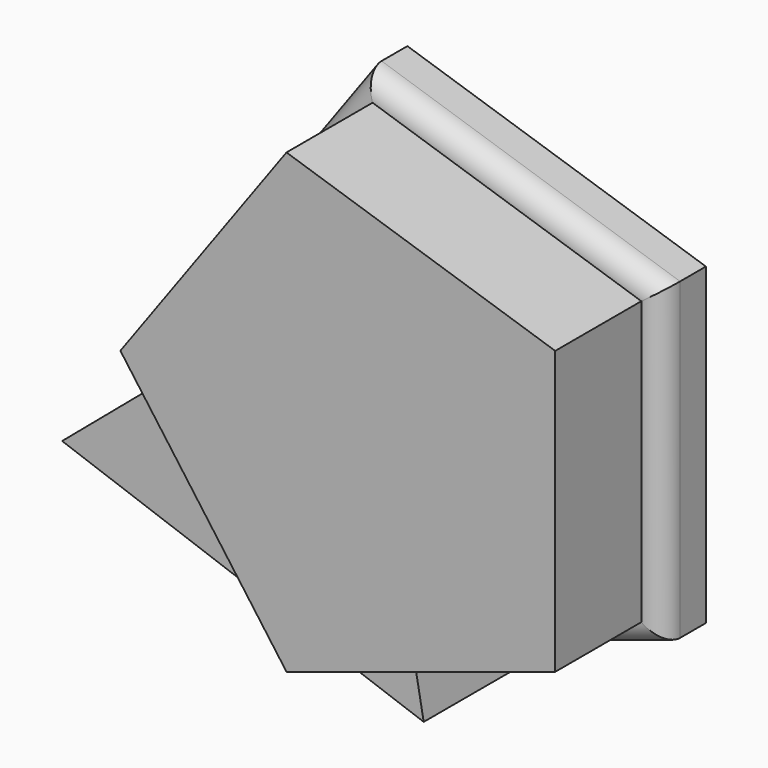
from build123d import *

# Parameters (mm, degrees)
F1_DEPTH     = 12.7
F2_R         = 5.08
F3_TEXT_SIZE = 35.0921052612
F4_DEPTH     = 25.4
F6_DEPTH     = 25.4


# Not quite as in the source:
# - Text() gives the source's letters only with a copy of the font that has no kerning and outlines rounded to 1/6400 em; it was checked with that copy


with BuildPart() as f1:
    # F0 (on Front) → F1 (new body)
    with BuildSketch(Plane.XZ):
        Polygon((50.9689189494, -37.0310872232), (50.9689189494, 37.0310872232), (-19.4683946688, 59.9175577675), (-63.0010485611, 0), (-19.4683946688, -59.9175577675), align=None)
    extrude(amount=F1_DEPTH)

    # F2
    f2_edges = [f1.edges().sort_by_distance(p)[0] for p in [
        (15.750262, -12.7, -48.474322),
        (50.968919, -12.7, 0),
        (15.750262, -12.7, 48.474322),
        (-41.234722, -12.7, 29.958779),
        (-41.234722, -12.7, -29.958779),
    ]]
    fillet(f2_edges, radius=F2_R)

    # F1_face (on face) + F3 (on Front) → F4 (join)
    with BuildSketch(Plane.XZ.offset(12.7)):
        Polygon((-17.5280073317, -53.9456596042), (45.8889189494, -33.3402511809), (45.8889189494, 33.3402511809), (-17.5280073317, 53.9456596042), (-56.7218232354, 0), align=None)
    with BuildSketch(Plane.XZ):
        with Locations((-42.2084573656, -12.1435001493)):
            Text('D&M', F3_TEXT_SIZE, font='Open Sans', font_style=FontStyle.BOLD, text_align=(TextAlign.LEFT, TextAlign.BOTTOM))
    extrude(amount=F4_DEPTH)

    # F5 (on Front) → F6 (join)
    with BuildSketch(Plane.XZ):
        Polygon((4.6952606254, -62.3020479672), (-11.4635487163, 26.9001076214), (-80.6354768574, -31.6949095577), align=None)
    extrude(amount=F6_DEPTH)


solid = f1.part
